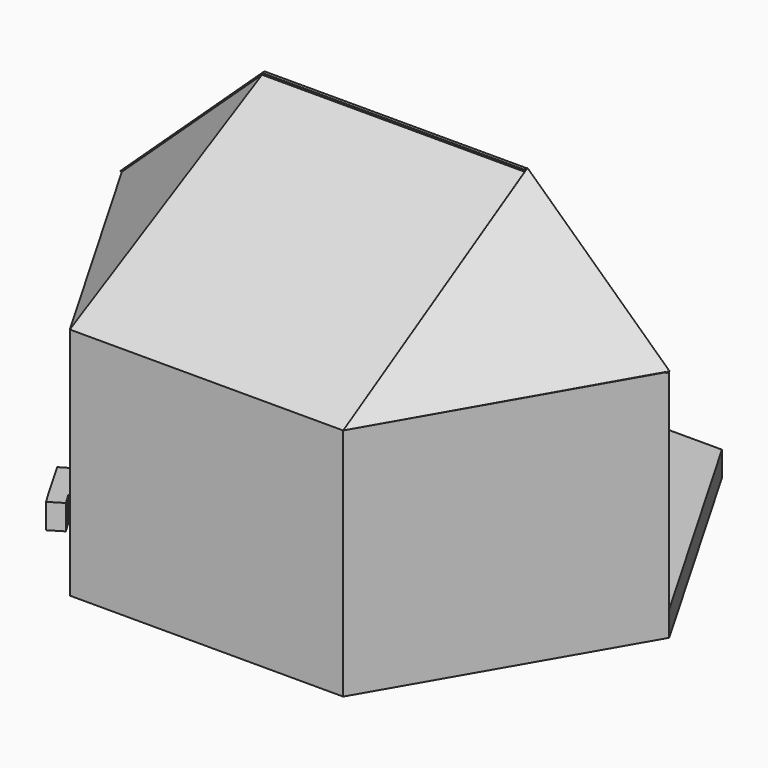
from build123d import *

# Parameters (mm, degrees)
F0_W      = 50
F0_H      = 12.5
F1_DEPTH  = 8
F2_DEPTH  = 75
F4_DEPTH  = 8
F7_DEPTH  = 3
F8_DEPTH  = 1
F11_DEPTH = 3
F14_DEPTH = 3
F15_DEPTH = 8
F16_DEPTH = 8
F17_DEPTH = 12.5


# Not quite as in the source:
# - a feature names something its author has since deleted; it is built from what else it names


with BuildPart() as f1:
    # F0 (on Top) → F1 (new body)
    with BuildSketch(Plane.XY):
        Polygon((42.0179491924, -72.7772228311), (84.0358983849, 0), (42.0179491924, 72.7772228311), (-42.0179491924, 72.7772228311), (-84.0358983849, 0), (-42.0179491924, -72.7772228311), align=None)
        with Locations((0, 54.5829171234)):
            Rectangle(F0_W, F0_H, mode=Mode.SUBTRACT)
    extrude(amount=F1_DEPTH)

    # F0 (on Top) → F2 (join)
    with BuildSketch(Plane.XY):
        Polygon((43.75, -75.7772228311), (87.5, 0), (84.0358983849, 0), (42.0179491924, -72.7772228311), (-42.0179491924, -72.7772228311), (-84.0358983849, 0), (-87.5, 0), (-68.1246734519, -33.5590499945), (-63.1805508476, -42.1225215441), (-43.75, -75.7772228311), align=None)
    extrude(amount=F2_DEPTH)

    # F0 (on Top) → F4 (join)
    with BuildSketch(Plane.XY):
        Polygon((43.75, 75.7772228311), (-43.75, 75.7772228311), (-65.625, 37.8886114156), (-68.125, 33.5584843966), (-87.5, 0), (-84.0358983849, 0), (-42.0179491924, 72.7772228311), (42.0179491924, 72.7772228311), (84.0358983849, 0), (87.5, 0), align=None)
    extrude(amount=F4_DEPTH)

    # F6 (on face) → F7 (join)
    with BuildSketch(Plane(origin=(0, -50.1312366318, 89.3836679776), x_dir=(1, 0, 0), z_dir=(0, 0.4891706574, -0.872188092))):
        Polygon((43.75, 29.4041920927), (0, 29.4041920927), (-43.75, 29.4041920927), (-42.01795, -57.4775522498), (42.01795, -57.4775522498), align=None)
    extrude(amount=F7_DEPTH)

    # F3 (on Front) → F8 (join)
    with BuildSketch(Plane.XZ):
        Polygon((-42.01795, 114.5), (0, 114.5), (42.01795, 114.5), (84.0359, 75), (87.5, 75), (42.01795, 117.5), (0, 117.5), (-42.01795, 117.5), (-87.5, 75), (-84.0359, 75), align=None)
    extrude(amount=F8_DEPTH)

    # F10 (on face) → F11 (join)
    with BuildSketch(Plane(origin=(-67.6846727043, -39.0777640058, 72.4338274863), x_dir=(0.7723629594, -0.3015876344, 0.5590173143), z_dir=(-0.6351814378, -0.3667221741, 0.6797495039))):
        Polygon((33.2314262259, 55.789645187), (-25.6554603702, 35.6104118215), (30.9888924807, -31.0804218073), align=None)
    extrude(amount=-F11_DEPTH)

    # F13 (on face) → F14 (join)
    with BuildSketch(Plane(origin=(67.6756688636, -39.5950852503, 72.4241918832), x_dir=(0.7733047167, 0.3041472681, -0.556322078), z_dir=(-0.6340345536, 0.3709553614, -0.6785221475))):
        Polygon((-30.939509805, 30.5117392321), (-32.8751652468, -56.3649154418), (25.9400068576, -35.9776056011), align=None)
    extrude(amount=F14_DEPTH)

    # F0 (on Top) → F15 (join)
    with BuildSketch(Plane.XY):
        with Locations((0, 54.5829171234)):
            Rectangle(F0_W, F0_H)
    extrude(amount=F15_DEPTH)

    # F0 (on Top) → F16 (join)
    with BuildSketch(Plane.XY):
        Polygon((-77.8456263738, -39.3203930924), (-73.5443197712, -36.7711262349), (-75.7943197712, -32.8740119179), (-80.0956263738, -35.4232787754), align=None)
        Polygon((-63.1805508476, -42.1225215441), (-68.1246734519, -33.5590499945), (-73.5443197712, -36.7711262349), (-77.8456263738, -39.3203930924), (-72.8440428469, -47.9797326875), (-68.5681614313, -45.3880463409), align=None)
        Polygon((-66.2356437193, -49.236339615), (-68.5681614313, -45.3880463409), (-72.8440428469, -47.9797326875), (-70.5115251349, -51.8280259616), align=None)
    extrude(amount=F16_DEPTH)

    # F0 (on Top) → F17 (cut, symmetric)
    with BuildSketch(Plane.XY):
        with Locations((0, 54.5829171234)):
            Rectangle(F0_W, F0_H)
    extrude(amount=F17_DEPTH, both=True, mode=Mode.SUBTRACT)


solid = f1.part
